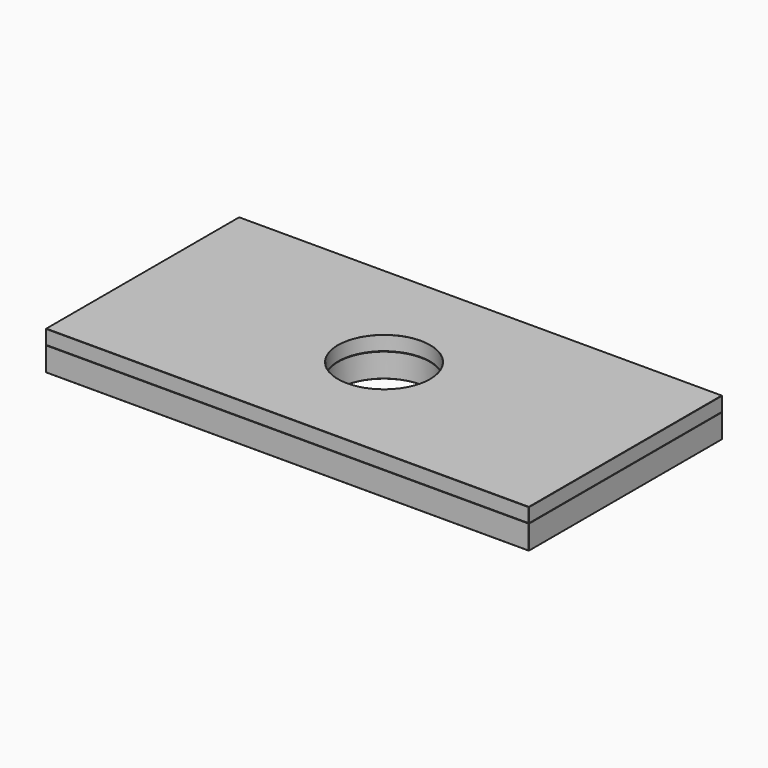
from build123d import *

# Parameters (mm, degrees)
F0_R      = 95
F1_DEPTH  = 50
F3_W      = 1000
F3_H      = 500
F3_W_2    = 920
F3_H_2    = 420
F3_R      = 95
F4_DEPTH  = 30
F5_SIZE   = 0.5
F6_D      = 10
F6_DEPTH  = 20
F6_TIP    = 3.0043030951
F7_SIZE   = 0.5
F7_2_SIZE = 0.5


# Not quite as in the source:
# - a feature names something its author has since deleted; it is built from what else it names


with BuildPart() as f1:
    # F0 (on Top) → F1 (new body)
    with BuildSketch(Plane.XY):
        with BuildLine():
            Line((330, 75), (350, 75))
            Line((350, 75), (350, 250))
            Line((350, 250), (-650, 250))
            Line((-650, 250), (-650, 75))
            Line((-650, 75), (-630, 75))
            ThreePointArc((-630, 75), (-622.9289321881, 72.0710678119), (-620, 65))
            Line((-620, 65), (-620, 0))
            Line((-620, 0), (-620, -65))
            ThreePointArc((-620, -65), (-622.9289321881, -72.0710678119), (-630, -75))
            Line((-630, -75), (-650, -75))
            Line((-650, -75), (-650, -250))
            Line((-650, -250), (350, -250))
            Line((350, -250), (350, -75))
            Line((350, -75), (330, -75))
            ThreePointArc((330, -75), (322.9289321881, -72.0710678119), (320, -65))
            Line((320, -65), (320, 65))
            ThreePointArc((320, 65), (322.9289321881, 72.0710678119), (330, 75))
        make_face()
        with Locations((-150, 0)):
            Circle(F0_R, mode=Mode.SUBTRACT)
        with BuildLine():
            Line((350, -75), (350, 75))
            Line((350, 75), (330, 75))
            ThreePointArc((330, 75), (322.9289321881, 72.0710678119), (320, 65))
            Line((320, 65), (320, -65))
            ThreePointArc((320, -65), (322.9289321881, -72.0710678119), (330, -75))
            Line((330, -75), (350, -75))
        make_face()
        with BuildLine():
            Line((-650, 0), (-650, -75))
            Line((-650, -75), (-630, -75))
            ThreePointArc((-630, -75), (-622.9289321881, -72.0710678119), (-620, -65))
            Line((-620, -65), (-620, 0))
            Line((-620, 0), (-650, 0))
        make_face()
        with BuildLine():
            Line((-630, 75), (-650, 75))
            Line((-650, 75), (-650, 0))
            Line((-650, 0), (-620, 0))
            Line((-620, 0), (-620, 65))
            ThreePointArc((-620, 65), (-622.9289321881, 72.0710678119), (-630, 75))
        make_face()
    extrude(amount=F1_DEPTH)

    # F7
    f7_edges = [f1.edges().sort_by_distance(p)[0] for p in [
        (-150, -250, 50),
        (350, 0, 50),
        (-150, 250, 50),
        (-650, 0, 50),
        (-245, 0, 50),
        (-650, -250, 25),
        (350, -250, 25),
        (-150, -250, 0),
        (350, 250, 25),
        (-650, 250, 25),
        (-150, 250, 0),
        (350, 0, 0),
        (-650, 0, 0),
        (-245, 0, 0),
    ]]
    chamfer(f7_edges, length=F7_SIZE)


with BuildPart() as f4:
    # F3 (on face) → F4 (new body)
    with BuildSketch(Plane.XY.offset(50)):
        with Locations((-150, 0)):
            Rectangle(F3_W, F3_H)
        with Locations((-150, 0)):
            Rectangle(F3_W_2, F3_H_2, mode=Mode.SUBTRACT)
        with Locations((-150, 0)):
            Rectangle(F3_W_2, F3_H_2)
        with Locations((-150, 0)):
            Circle(F3_R, mode=Mode.SUBTRACT)
    extrude(amount=F4_DEPTH)

    # F5
    f5_edges = [f4.edges().sort_by_distance(p)[0] for p in [
        (-150, 250, 80),
        (-650, 0, 80),
        (-150, -250, 80),
        (350, 0, 80),
        (-245, 0, 80),
        (-150, 250, 50),
        (-650, 0, 50),
        (-150, -250, 50),
        (350, 0, 50),
        (-245, 0, 50),
        (350, 250, 65),
        (-650, 250, 65),
        (-650, -250, 65),
        (350, -250, 65),
    ]]
    chamfer(f5_edges, length=F5_SIZE)

    # F6
    with Locations(Plane(origin=(0, 0, 50), x_dir=(1, 0, 0), z_dir=(0, 0, -1))):
        with Locations((-610, -210), (310, -210), (310, 210), (-610, 210)):
            Hole(F6_D / 2, depth=F6_DEPTH)
            with Locations((0, 0, -(F6_DEPTH + F6_TIP / 2))):  # 118° drill point
                Cone(0, F6_D / 2, F6_TIP, mode=Mode.SUBTRACT)

    # F7#2
    f7_2_edges = [f4.edges().sort_by_distance(p)[0] for p in [
        (-245, 0, 79.5),
    ]]
    chamfer(f7_2_edges, length=F7_2_SIZE)


solid = Compound([f1.part, f4.part])
